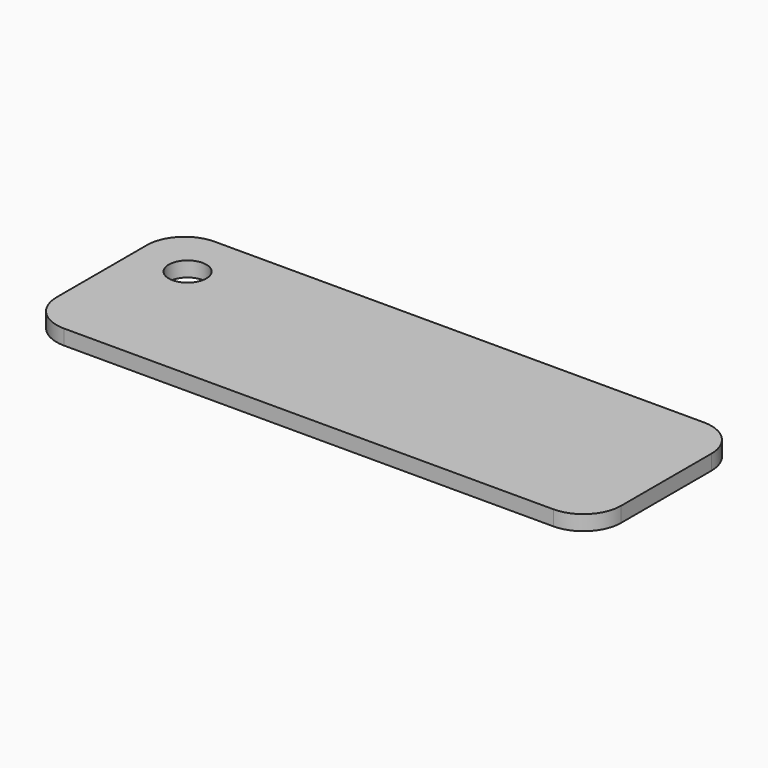
from build123d import *

# Parameters (mm, degrees)
F1_DEPTH     = 2
F3_D         = 5
F4_TEXT_SIZE = 15.4166676415
F5_DEPTH     = 1


# Not quite as in the source:
# - Text() gives the source's letters only with a copy of the font that has no kerning and outlines rounded to 1/6400 em; it was checked with that copy


with BuildPart() as f1:
    # F0 (on Top) → F1 (new body)
    with BuildSketch(Plane.XY):
        with BuildLine():
            ThreePointArc((37.5, 7.5), (36.0355339059, 11.0355339059), (32.5, 12.5))
            Line((32.5, 12.5), (-32.5, 12.5))
            ThreePointArc((-32.5, 12.5), (-36.0355339059, 11.0355339059), (-37.5, 7.5))
            Line((-37.5, 7.5), (-37.5, -7.5))
            ThreePointArc((-37.5, -7.5), (-36.0355339059, -11.0355339059), (-32.5, -12.5))
            Line((-32.5, -12.5), (32.5, -12.5))
            ThreePointArc((32.5, -12.5), (36.0355339059, -11.0355339059), (37.5, -7.5))
            Line((37.5, -7.5), (37.5, 7.5))
        make_face()
    extrude(amount=F1_DEPTH)

    # F3 (through all)
    with Locations(Plane(origin=(0, 0, 0), x_dir=(1, 0, 0), z_dir=(0, 0, -1))):
        with Locations((-30.5, -5.5)):
            Hole(F3_D / 2)

    # F4 (on Top) → F5 (join)
    with BuildSketch(Plane.XY):
        with Locations((-18.1499999017, 0)):
            Text('Torin', F4_TEXT_SIZE, font='Open Sans', text_align=(TextAlign.LEFT, TextAlign.BOTTOM))
    extrude(amount=F5_DEPTH)


solid = f1.part
